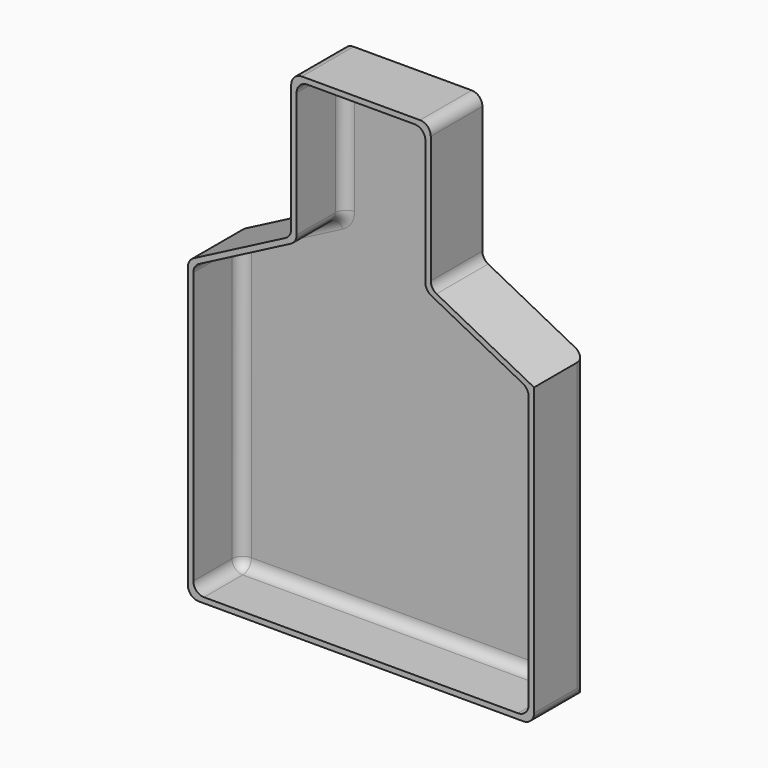
from build123d import *

# Parameters (mm, degrees)
F1_DEPTH = 30
F2_T     = -2.5
F3_R     = 5
F4_R     = 5


with BuildPart() as f1:
    # F0 (on Front) → F1 (new body)
    with BuildSketch(Plane.XZ):
        Polygon((-80.4619731335, 48.0414940363), (-80.4619731335, -90.2443051724), (80.4619731335, -90.2443051724), (80.4619731335, 48.0414940363), (32.4382460701, 72.9859998765), (32.4382460701, 140.1879998765), (-32.4382460701, 140.1879998765), (-32.4382460701, 72.9859998765), align=None)
    extrude(amount=F1_DEPTH)

    # F2
    f2_openings = [f1.faces().sort_by_distance(p)[0] for p in [
        (0, -30, 5.455809),
    ]]
    offset(amount=F2_T, openings=f2_openings, kind=Kind.INTERSECTION)

    # F3
    f3_edges = [f1.edges().sort_by_distance(p)[0] for p in [
        (-77.961973, -2.5, -20.610696),
        (-53.95011, -2.5, 58.995166),
        (-29.938246, -2.5, 104.577709),
        (0, -2.5, 137.688),
        (29.938246, -16.25, 137.688),
        (29.938246, -2.5, 104.577709),
        (53.95011, -2.5, 58.995166),
        (29.938246, -16.25, 71.467419),
        (-29.938246, -16.25, 71.467419),
        (-77.961973, -16.25, -87.744305),
        (0, -2.5, -87.744305),
        (77.961973, -16.25, -87.744305),
        (77.961973, -2.5, -20.610696),
        (-77.961973, -16.25, 46.522913),
        (-29.938246, -16.25, 137.688),
        (77.961973, -16.25, 46.522913),
    ]]
    fillet(f3_edges, radius=F3_R)

    # F4
    f4_edges = [f1.edges().sort_by_distance(p)[0] for p in [
        (32.438246, -15, 140.188),
        (80.461973, 0, -21.101406),
        (-32.438246, -15, 140.188),
        (-32.438246, -15, 72.986),
        (32.438246, -15, 72.986),
        (-80.461973, -15, 48.041494),
        (-80.461973, -15, -90.244305),
        (80.461973, -15, -90.244305),
    ]]
    fillet(f4_edges, radius=F4_R)


solid = f1.part
